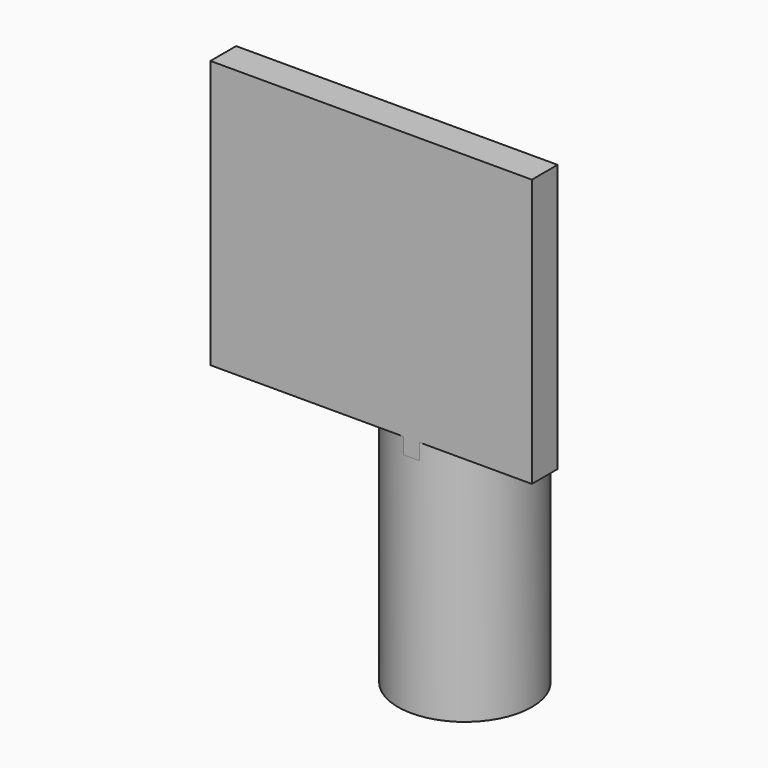
from build123d import *

# Parameters (mm, degrees)
F0_W         = 60
F0_H         = 50
F1_DEPTH     = 6
F2_R         = 12.5
F3_DEPTH     = 6
F4_W         = 3
F4_H         = 20
F5_DEPTH     = 3
F6_R         = 12.5
F7_DEPTH     = 45
F8_R         = 1.75
F9_DEPTH     = 51.001
F10_T1_DEPTH = 6
F11_R        = 10
F12_DEPTH    = 3


# Not quite as in the source:
# - a fillet or chamfer that OpenCascade refuses, or shapes differently, is made with other operations: its cross-section is extruded or revolved along the edge and cut away or added


with BuildPart() as f1:
    # F0 (on Front) → F1 (new body)
    with BuildSketch(Plane.XZ):
        with Locations((-30, 25)):
            Rectangle(F0_W, F0_H)
    extrude(amount=F1_DEPTH)

    # F2 (on face) → F3 (join)
    with BuildSketch(Plane(origin=(0, 0, 0), x_dir=(1, 0, 0), z_dir=(0, 0, -1))):
        with Locations((-22.5, -6.5)):
            Circle(F2_R)
    extrude(amount=-F3_DEPTH)

    # F4 (on face) → F5 (join)
    with BuildSketch(Plane(origin=(0, 0, 0), x_dir=(1, 0, 0), z_dir=(0, 0, -1))):
        with Locations((-22.5, -4)):
            Rectangle(F4_W, F4_H)
    extrude(amount=F5_DEPTH)


with BuildPart() as f7:
    # F6 (on face) → F7 (new body)
    with BuildSketch(Plane(origin=(0, 0, 0), x_dir=(1, 0, 0), z_dir=(0, 0, -1))):
        with Locations((-22.5, -6.5)):
            Circle(F6_R)
    extrude(amount=F7_DEPTH)


with BuildPart() as f9_tool:
    # F8 (on face) → F9 (new body, through all)
    with BuildSketch(Plane.XY.offset(6)):
        with Locations((-22.5, 6.5)):
            Circle(F8_R)
    extrude(amount=-F9_DEPTH)


with BuildPart() as f1_1:
    add(f1.part)

    # F9: cut by f9_tool
    add(f9_tool.part, mode=Mode.SUBTRACT)

    # F10: fillet of radius 35 on 2 edges, made by hand

    # F10_s2 → F10_t1 (join)
    with BuildSketch(Plane.XY):
        with BuildLine():
            ThreePointArc((-59.9999942526, -0.0003999587), (-44.6241465011, 3.8051050521), (-32.5003627011, 13.9988496455))
            Line((-32.5003627011, 13.9988496455), (-29.7001088019, 11.8990575092))
            ThreePointArc((-29.7001088019, 11.8990575092), (-31.4894392952, 6.9342461078), (-30.1874293614, 1.8200407762))
            Line((-30.1874293614, 1.8200407762), (-33.177078252, -3.5000784157))
            Line((-33.177078252, -3.5000784157), (-59.9497035085, -3.5001170554))
            Line((-59.9497035085, -3.5001170554), (-59.9999942526, -0.0003999587))
        make_face()
    extrude(amount=F10_T1_DEPTH)

    # F11
    f11_edges = [f1_1.edges().sort_by_distance(p)[0] for p in [
        (-11.822922, 0, 3),
    ]]
    fillet(f11_edges, radius=F11_R)


with BuildPart() as f7_1:
    add(f7.part)

    # F9: cut by f9_tool
    add(f9_tool.part, mode=Mode.SUBTRACT)

    # F4 (on face) → F12 (cut)
    with BuildSketch(Plane(origin=(0, 0, 0), x_dir=(1, 0, 0), z_dir=(0, 0, -1))):
        with Locations((-22.5, -4)):
            Rectangle(F4_W, F4_H)
    extrude(amount=F12_DEPTH, mode=Mode.SUBTRACT)


solid = Compound([f1_1.part, f7_1.part])
